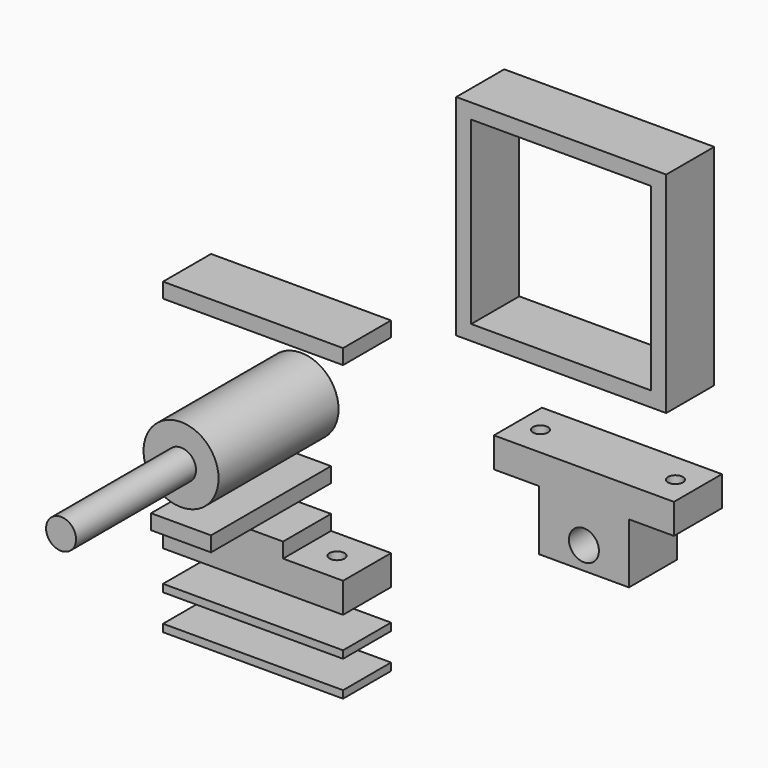
from build123d import *

# Parameters (mm, degrees)
F0_R      = 5
F1_DEPTH  = 20
F0_W      = 60
F0_H      = 5
F0_W_2    = 70
F0_H_2    = 70
F0_H_3    = 60
F0_H_4    = 2.5
F0_R_2    = 12.5
F2_DEPTH  = 50
F3_R      = 5
F4_DEPTH  = 50
F5_DEPTH  = 50
F6_R      = 2.5
F7_R      = 2.5
F8_DEPTH  = 25
F10_R     = 2.5
F9_R      = 2.5
F11_DEPTH = 25


# Not quite as in the source:
# - a feature of the source that left no trace in its solid (it failed there, or was rolled back) is left out


with BuildPart() as f1:
    # F0 (on Front) → F1 (new body)
    with BuildSketch(Plane.XZ):
        Polygon((95.2936565876, -7.5), (110.2936565876, -7.5), (125.2936565876, -7.5), (125.2936565876, 12.5), (140.2936565876, 12.5), (140.2936565876, 22.5), (110.2936565876, 22.5), (80.2936565876, 22.5), (80.2936565876, 12.5), (95.2936565876, 12.5), align=None)
        with Locations((110.2936565876, 0)):
            Circle(F0_R, mode=Mode.SUBTRACT)
    extrude(amount=F1_DEPTH)

    # F10 (on face) + F9 (on face) → F11 (cut)
    with BuildSketch(Plane(origin=(0, 0, 12.5), x_dir=(1, 0, 0), z_dir=(0, 0, -1))):
        with Locations((87.7936565876, 10)):
            Circle(F10_R)
    with BuildSketch(Plane(origin=(0, 0, 12.5), x_dir=(1, 0, 0), z_dir=(0, 0, -1))):
        with Locations((132.7936565876, 10)):
            Circle(F9_R)
    extrude(amount=-F11_DEPTH, mode=Mode.SUBTRACT)


with BuildPart() as f1b:
    # F0 (on Front) → F1, piece 2 (new body)
    with BuildSketch(Plane.XZ):
        with Locations((0, 29.2427036911)):
            Rectangle(F0_W, F0_H)
    extrude(amount=F1_DEPTH)


with BuildPart() as f1c:
    # F0 (on Front) → F1, piece 3 (new body)
    with BuildSketch(Plane.XZ):
        Polygon((10, -31.5313972533), (0, -31.5313972533), (-10, -31.5313972533), (-10, -36.5313972533), (-30, -36.5313972533), (-30, -46.5313972533), (0, -46.5313972533), (30, -46.5313972533), (30, -36.5313972533), (10, -36.5313972533), align=None)
    extrude(amount=F1_DEPTH)

    # F6 (on face) + F7 (on face) → F8 (cut)
    with BuildSketch(Plane.XY.offset(-36.5313972533)):
        with Locations((-20, -10)):
            Circle(F6_R)
    with BuildSketch(Plane.XY.offset(-36.5313972533)):
        with Locations((20, -10)):
            Circle(F7_R)
    extrude(amount=-F8_DEPTH, mode=Mode.SUBTRACT)


with BuildPart() as f1d:
    # F0 (on Front) → F1, piece 4 (new body)
    with BuildSketch(Plane.XZ):
        with Locations((102.7326732874, 82.7068325877)):
            Rectangle(F0_W_2, F0_H_2)
        with Locations((102.7326732874, 82.7068325877)):
            Rectangle(F0_W, F0_H_3, mode=Mode.SUBTRACT)
    extrude(amount=F1_DEPTH)


with BuildPart() as f1e:
    # F0 (on Front) → F1, piece 5 (new body)
    with BuildSketch(Plane.XZ):
        with Locations((0, -58.184633702)):
            Rectangle(F0_W, F0_H_4)
    extrude(amount=F1_DEPTH)


with BuildPart() as f1f:
    # F0 (on Front) → F1, piece 6 (new body)
    with BuildSketch(Plane.XZ):
        with Locations((0, -69.8959429562)):
            Rectangle(F0_W, F0_H_4)
    extrude(amount=F1_DEPTH)


with BuildPart() as f2:
    # F0 (on Front) → F2 (new body)
    with BuildSketch(Plane.XZ):
        Circle(F0_R_2)
    extrude(amount=F2_DEPTH)

    # F3 (on face) → F4 (join)
    with BuildSketch(Plane.XZ.offset(50)):
        Circle(F3_R)
    extrude(amount=F4_DEPTH)


with BuildPart() as f5:
    # F0 (on Front) → F5 (new body)
    with BuildSketch(Plane.XZ):
        Polygon((-10, -22.5167013705), (0, -22.5167013705), (10, -22.5167013705), (10, -17.5167013705), (0, -17.5167013705), (-10, -17.5167013705), align=None)
    extrude(amount=F5_DEPTH)


solid = Compound([f1.part, f1b.part, f1c.part, f1d.part, f1e.part, f1f.part, f2.part, f5.part])
